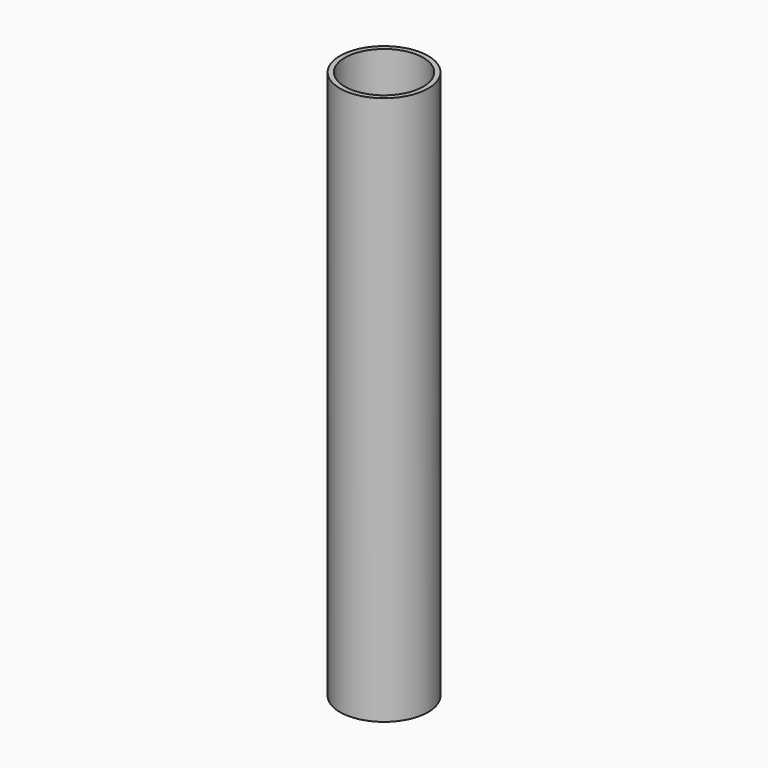
from build123d import *

# Parameters (mm, degrees)
F0_R     = 14.2875
F0_R_2   = 12.7
F1_DEPTH = 177.8


# Not quite as in the source:
# - a feature names something its author has since deleted; it is built from what else it names


with BuildPart() as f1:
    # F0 (on Top) → F1 (new body)
    with BuildSketch(Plane.XY):
        Circle(F0_R)
        Circle(F0_R_2, mode=Mode.SUBTRACT)
    extrude(amount=F1_DEPTH)


solid = f1.part
